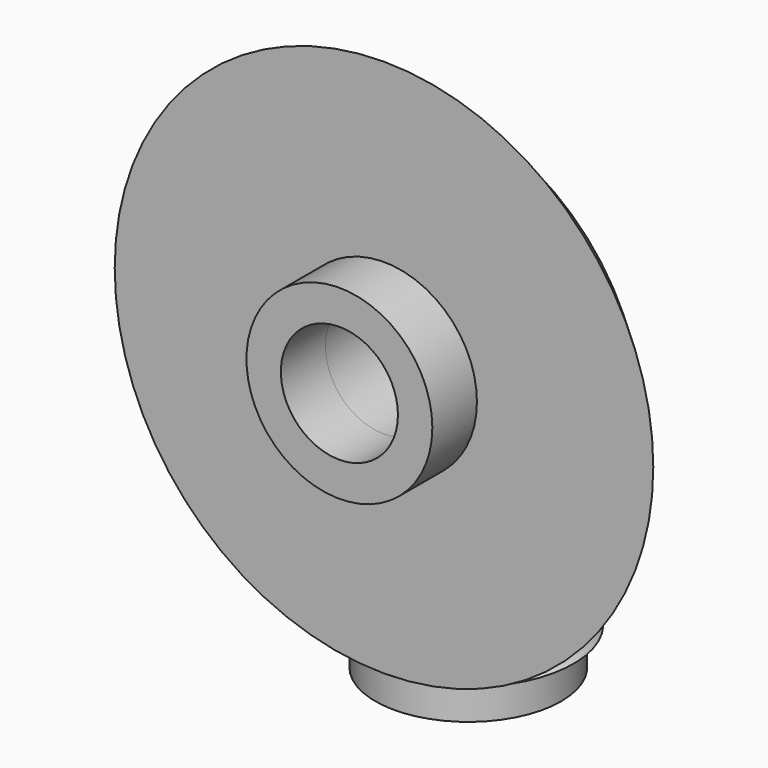
from build123d import *
from build123d import SkipClean  # not in build123d's __all__

# Parameters (mm, degrees)
F3_R          = 5
F4_DEPTH      = 7.621
F5_R          = 4
F6_DEPTH      = 46.001
F7_W          = 8
F7_H          = 36
F8_DEPTH      = 23.0010001
F8_DEPTH_BACK = 23.0010001
F9_R          = 7.9375
F9_R_2        = 4
F10_DEPTH     = 3.175
F11_R         = 7.9375
F11_R_2       = 5
F12_DEPTH     = 4.7625


with BuildPart() as f1:
    # F0 (on Right) → F1 (revolve)
    with BuildSketch(Plane.YZ):
        Polygon((-1.38, 0), (-9, 0), (-9, -23), (-1.38, -15.38), align=None)
    revolve(axis=Axis((0, -5.19, 0), (0, 1, 0)))

    # F3 (on face) → F4 (cut, through all)
    with BuildSketch(Plane(origin=(0, -1.38, 0), x_dir=(-1, 0, 0), z_dir=(0, 1, 0))):
        Circle(F3_R)
    extrude(amount=-F4_DEPTH, mode=Mode.SUBTRACT)


with BuildPart() as f2:
    # F0 (on Right) → F2 (revolve)
    with BuildSketch(Plane.YZ):
        Polygon((-1.38, -15.38), (-9, -23), (0, -23), (0, -15.38), align=None)
    revolve(axis=Axis((0, 0, -19.19), (0, 0, -1)))


with BuildPart() as f6_tool:
    # F5 (on face) → F6 (new body, through all)
    with BuildSketch(Plane(origin=(0, 0, -23), x_dir=(1, 0, 0), z_dir=(0, 0, -1))):
        Circle(F5_R)
    extrude(amount=-F6_DEPTH)


with BuildPart() as f1_1:
    add(f1.part, clean=False)

    # F6: cut by f6_tool
    add(f6_tool.part, mode=Mode.SUBTRACT)

    # F7 (on Right) → F8 (cut, two sides)
    with BuildSketch(Plane.YZ) as f8_sk:
        Rectangle(F7_W, F7_H)
    extrude(amount=-F8_DEPTH, mode=Mode.SUBTRACT)
    extrude(f8_sk.sketch, amount=F8_DEPTH_BACK, mode=Mode.SUBTRACT)

    # F11 (on face) → F12 (join)
    with BuildSketch(Plane.XZ.offset(9)):
        Circle(F11_R)
        Circle(F11_R_2, mode=Mode.SUBTRACT)
    with SkipClean():  # cleaning this boolean's faces spoils the solid; the shape is the same uncleaned
        extrude(amount=F12_DEPTH)


with BuildPart() as f2_1:
    add(f2.part, clean=False)

    # F6: cut by f6_tool
    add(f6_tool.part, mode=Mode.SUBTRACT)

    # F9 (on face) → F10 (join)
    with BuildSketch(Plane(origin=(0, 0, -23), x_dir=(1, 0, 0), z_dir=(0, 0, -1))):
        Circle(F9_R)
        Circle(F9_R_2, mode=Mode.SUBTRACT)
    extrude(amount=F10_DEPTH)


solid = Compound([f1_1.part, f2_1.part])
